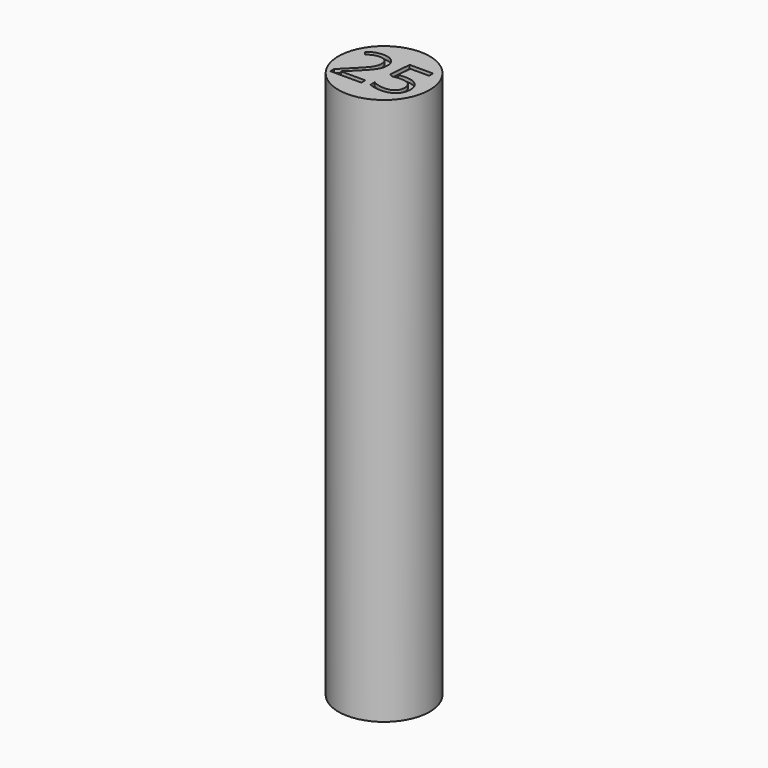
from build123d import *

# Parameters (mm, degrees)
F0_R         = 12.5
F1_DEPTH     = 150
F2_TEXT_SIZE = 18.0555555556
F3_DEPTH     = 1
F4_TEXT_SIZE = 18.0555555556
F5_DEPTH     = 1


# Not quite as in the source:
# - Text() gives the source's letters only with a copy of the font that has no kerning and outlines rounded to 1/6400 em; it was checked with that copy


with BuildPart() as f1:
    # F0 (on Top) → F1 (new body)
    with BuildSketch(Plane.XY):
        Circle(F0_R)
    extrude(amount=F1_DEPTH)

    # F2 (on face) → F3 (cut)
    with BuildSketch(Plane(origin=(0, 0, 0), x_dir=(1, 0, 0), z_dir=(0, 0, -1))):
        with Locations((-10.3889973958, -6.5)):
            Text('25', F2_TEXT_SIZE, font='Open Sans', text_align=(TextAlign.LEFT, TextAlign.BOTTOM))
    extrude(amount=-F3_DEPTH, mode=Mode.SUBTRACT)

    # F4 (on face) → F5 (cut)
    with BuildSketch(Plane.XY.offset(150)):
        with Locations((-10.3889973958, -6.5)):
            Text('25', F4_TEXT_SIZE, font='Open Sans', text_align=(TextAlign.LEFT, TextAlign.BOTTOM))
    extrude(amount=-F5_DEPTH, mode=Mode.SUBTRACT)


solid = f1.part
